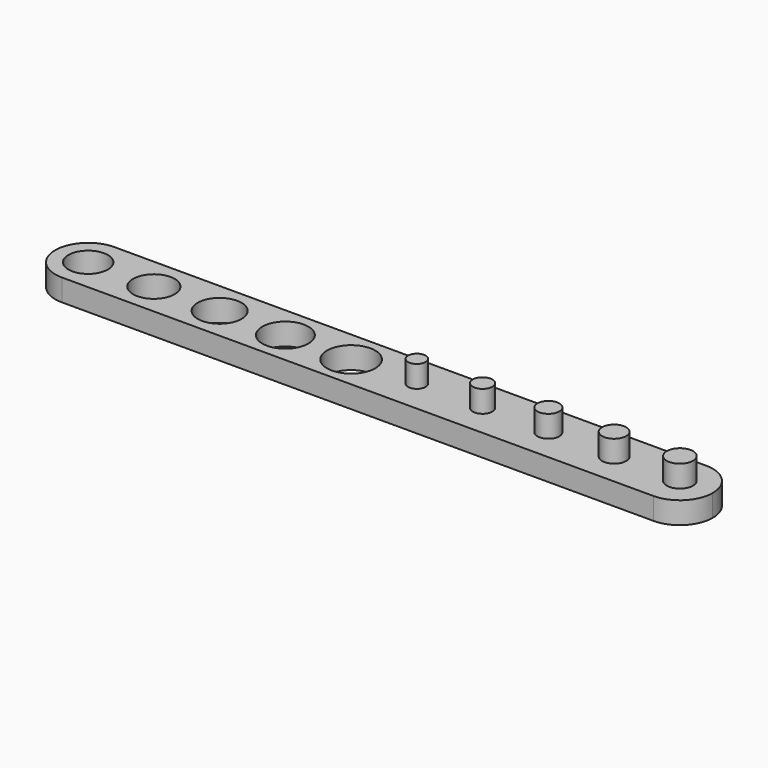
from build123d import *

# Parameters (mm, degrees)
F0_W     = 150
F0_H     = 15
F0_R     = 4.5
F0_R_2   = 4.75
F0_R_3   = 5
F0_R_4   = 5.25
F0_R_5   = 5.5
F1_DEPTH = 5
F2_R     = 7.49999
F3_R     = 3
F3_R_2   = 2.5
F3_R_3   = 2.75
F3_R_4   = 2.25
F3_R_5   = 2
F4_DEPTH = 10


# Not quite as in the source:
# - a fillet or chamfer is up to 0.001 mm smaller than in the source, because OpenCascade refuses the exact size


with BuildPart() as f1:
    # F0 (on Top) → F1 (new body)
    with BuildSketch(Plane.XY):
        Rectangle(F0_W, F0_H)
        with Locations((-67.5, 0)):
            Circle(F0_R, mode=Mode.SUBTRACT)
        with Locations((-52.5, 0)):
            Circle(F0_R_2, mode=Mode.SUBTRACT)
        with Locations((-37.5, 0)):
            Circle(F0_R_3, mode=Mode.SUBTRACT)
        with Locations((-22.5, 0)):
            Circle(F0_R_4, mode=Mode.SUBTRACT)
        with Locations((-7.5, 0)):
            Circle(F0_R_5, mode=Mode.SUBTRACT)
    extrude(amount=F1_DEPTH)

    # F2 (radius 7.5 in the source; OpenCascade refuses exactly that, so slightly less here)
    f2_edges = [f1.edges().sort_by_distance(p)[0] for p in [
        (-75, -7.5, 2.5),
        (-75, 7.5, 2.5),
        (75, -7.5, 2.5),
        (75, 7.5, 2.5),
    ]]
    fillet(f2_edges, radius=F2_R)

    # F3 (on Top) → F4 (join)
    with BuildSketch(Plane.XY):
        with Locations((67.5, 0)):
            Circle(F3_R)
        with Locations((37.5, 0)):
            Circle(F3_R_2)
        with Locations((52.5, 0)):
            Circle(F3_R_3)
        with Locations((22.5, 0)):
            Circle(F3_R_4)
        with Locations((7.5, 0)):
            Circle(F3_R_5)
    extrude(amount=F4_DEPTH)


solid = f1.part
